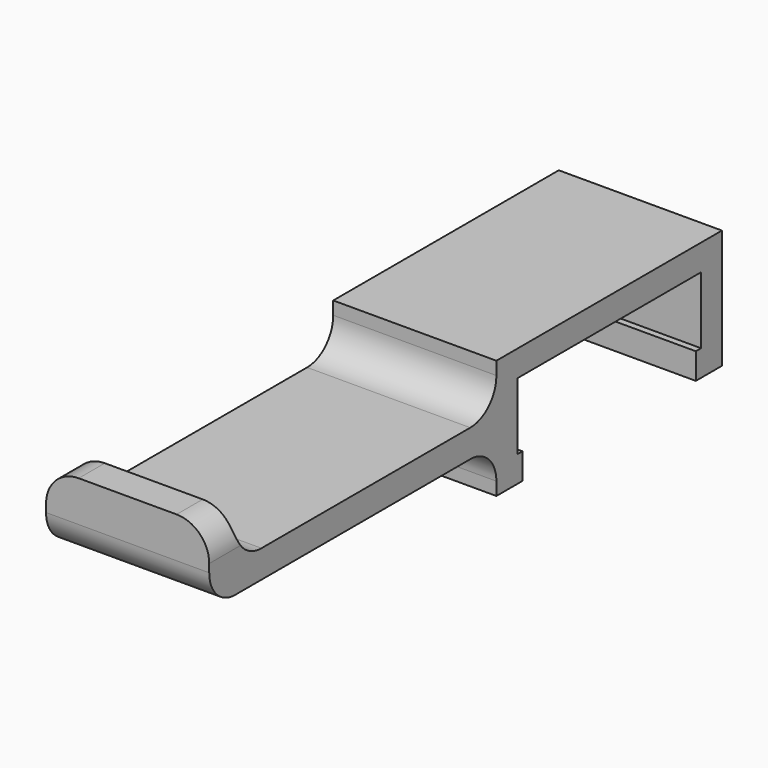
from build123d import *

# Parameters (mm, degrees)
F1_DEPTH = 25
F3_W     = 25
F3_H     = 4.25
F4_DEPTH = 55
F5_W     = 25
F5_H     = 5
F6_DEPTH = 7
F7_R     = 5
F8_R     = 5


# Not quite as in the source:
# - a feature of the source that left no trace in its solid (it failed there, or was rolled back) is left out


with BuildPart() as f1:
    # F0 (on Right) → F1 (new body)
    with BuildSketch(Plane.YZ):
        Polygon((17.6, 0.1), (17.6, -10.15), (16.6, -10.15), (16.6, -14.15), (21.6, -14.15), (21.6, 4.1), (0, 4.1), (-21.6, 4.1), (-21.6, -14.15), (-16.6, -14.15), (-16.6, -10.15), (-17.6, -10.15), (-17.6, 0.1), (0, 0.1), align=None)
    extrude(amount=F1_DEPTH)

    # F3 (on face) → F4 (join)
    with BuildSketch(Plane.XZ.offset(21.6)):
        with Locations((12.5, -5.025)):
            Rectangle(F3_W, F3_H)
    extrude(amount=F4_DEPTH)

    # F5 (on face) → F6 (join, through all)
    with BuildSketch(Plane.XY.offset(-2.9)):
        with Locations((12.5, -74.1)):
            Rectangle(F5_W, F5_H)
    extrude(amount=F6_DEPTH)

    # F7
    f7_edges = [f1.edges().sort_by_distance(p)[0] for p in [
        (12.5, -21.6, -2.9),
        (12.5, -21.6, -7.15),
        (12.5, -71.6, -2.9),
        (12.5, -76.6, -7.15),
    ]]
    fillet(f7_edges, radius=F7_R)

    # F8
    f8_edges = [f1.edges().sort_by_distance(p)[0] for p in [
        (0, -74.1, 4.1),
        (25, -74.1, 4.1),
    ]]
    fillet(f8_edges, radius=F8_R)


solid = f1.part
